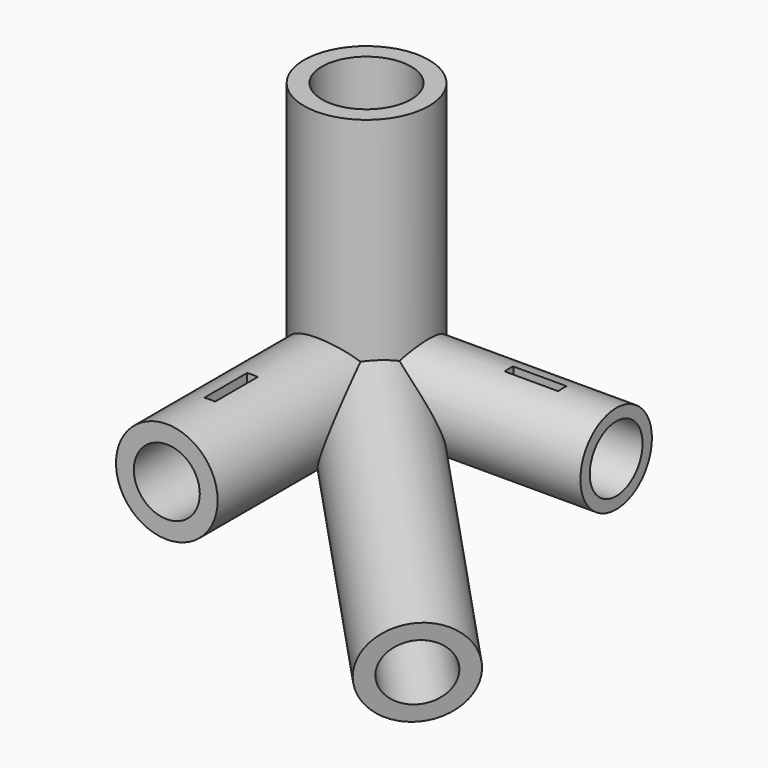
from build123d import *
from build123d import SkipClean  # not in build123d's __all__

# Parameters (mm, degrees)
F6_R      = 17.5
F6_R_2    = 12.5
F7_DEPTH  = 70
F8_R      = 14.25
F8_R_2    = 9.25
F9_DEPTH  = 70
F10_R     = 12.5291030152
F10_R_2   = 9.25
F11_DEPTH = 70
F15_R     = 14.25
F15_R_2   = 9.25
F16_DEPTH = 105
F19_DEPTH = 50
F20_DEPTH = 51
F21_DEPTH = 50
F22_DEPTH = 50
F6_W      = 15
F6_H      = 3
F27_DEPTH = 23.5
F6_W_2    = 3
F6_H_2    = 15
F28_DEPTH = 23.5


# Not quite as in the source:
# - a feature of the source that left no trace in its solid (it failed there, or was rolled back) is left out
# - a feature names something its author has since deleted; it is built from what else it names


with BuildPart() as f7:
    # F6 (on Top) → F7 (new body)
    with BuildSketch(Plane.XY):
        Circle(F6_R)
        Circle(F6_R_2, mode=Mode.SUBTRACT)
    extrude(amount=F7_DEPTH)

    # F8 (on Front) → F9 (join)
    with BuildSketch(Plane.XZ):
        Circle(F8_R)
        Circle(F8_R_2, mode=Mode.SUBTRACT)
    extrude(amount=F9_DEPTH)

    # F10 (on Right) → F11 (join)
    with BuildSketch(Plane.YZ):
        Circle(F10_R)
        Circle(F10_R_2, mode=Mode.SUBTRACT)
    extrude(amount=F11_DEPTH)

    # F15 (on face) → F16 (join)
    with BuildSketch(Plane(origin=(-1.0170364822, 1.0170364822, 0.3320592861), x_dir=(0.7247768542, 0.6549581555, 0.2138418251), z_dir=(0.6889836802, -0.6889836802, -0.2249510543))):
        Circle(F15_R)
        Circle(F15_R_2, mode=Mode.SUBTRACT)
    extrude(amount=F16_DEPTH)

    # F17 (on Top) → F18 (revolve, cut)
    with BuildSketch(Plane.XY):
        with BuildLine():
            Line((0, 17.5), (0, -17.5))
            ThreePointArc((0, -17.5), (17.5, 0), (0, 17.5))
        make_face()
    revolve(axis=Axis((0, 0, 0), (0, 1, 0)), mode=Mode.SUBTRACT)

    # F6 (on Top) → F19 (cut)
    with BuildSketch(Plane.XY):
        Circle(F6_R_2)
    extrude(amount=F19_DEPTH, mode=Mode.SUBTRACT)

    # F8 (on Front) → F20 (cut)
    with BuildSketch(Plane.XZ):
        Circle(F8_R_2)
    extrude(amount=F20_DEPTH, mode=Mode.SUBTRACT)

    # F15 (on face) → F21 (cut)
    with BuildSketch(Plane(origin=(-1.0170364822, 1.0170364822, 0.3320592861), x_dir=(0.7247768542, 0.6549581555, 0.2138418251), z_dir=(0.6889836802, -0.6889836802, -0.2249510543))):
        Circle(F15_R_2)
    with SkipClean():  # cleaning this boolean's faces spoils the solid; the shape is the same uncleaned
        extrude(amount=F21_DEPTH, mode=Mode.SUBTRACT)

    # F10 (on Right) → F22 (cut)
    with BuildSketch(Plane.YZ):
        Circle(F10_R_2)
    extrude(amount=F22_DEPTH, mode=Mode.SUBTRACT)

    # F17 (on Top) → F23 (revolve)
    with BuildSketch(Plane.XY):
        with BuildLine():
            Line((0, 17.5), (0, -17.5))
            ThreePointArc((0, -17.5), (17.5, 0), (0, 17.5))
        make_face()
    revolve(axis=Axis((0, 0, 0), (0, 1, 0)))

    # F6 (on Top) → F27 (cut)
    with BuildSketch(Plane.XY):
        with Locations((47.5, -0.0659547513)):
            Rectangle(F6_W, F6_H)
    extrude(amount=F27_DEPTH, mode=Mode.SUBTRACT)

    # F6 (on Top) → F28 (cut)
    with BuildSketch(Plane.XY):
        with Locations((0, -47.5)):
            Rectangle(F6_W_2, F6_H_2)
    extrude(amount=F28_DEPTH, mode=Mode.SUBTRACT)


solid = f7.part
